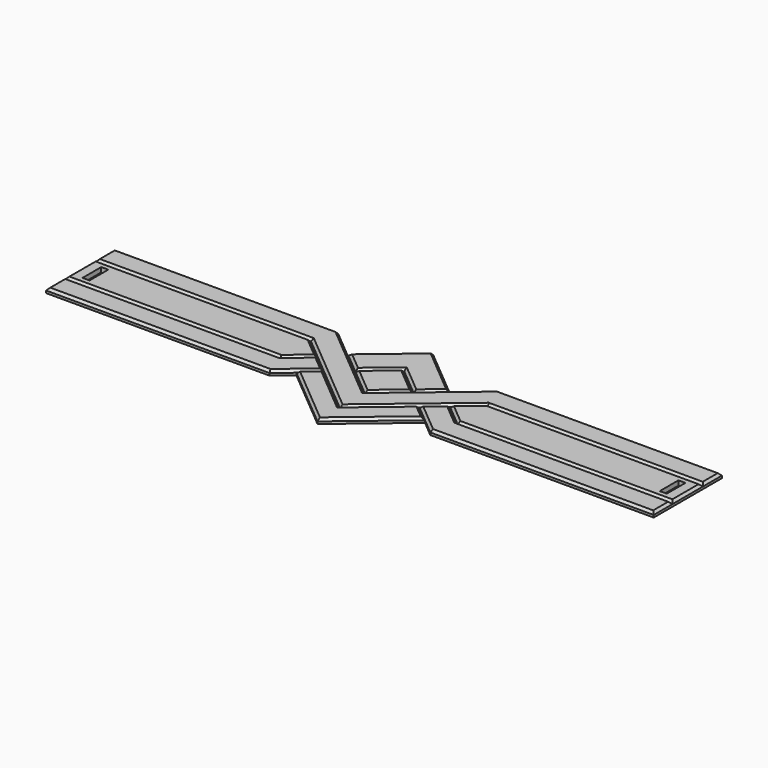
from build123d import *

# Parameters (mm, degrees)
F1_DEPTH  = 2
F3_DEPTH  = 2
F5_DEPTH  = 2
F7_DEPTH  = 2
F9_DEPTH  = 1
F10_SIZE  = 0.99999
F11_W     = 3
F11_H     = 10
F12_DEPTH = 2


# Not quite as in the source:
# - a fillet or chamfer is up to 0.001 mm smaller than in the source, because OpenCascade refuses the exact size


with BuildPart() as f1:
    # F0 (on Top) → F1 (new body)
    with BuildSketch(Plane.XY):
        Polygon((37.9150851114, 8), (28.3810563706, 0), (37.9150851114, -8), (130, -8), (130, 0), (130, 8), align=None)
    extrude(amount=F1_DEPTH)



with BuildPart() as f1b:
    # F0 (on Top) → F1, piece 2 (new body)
    with BuildSketch(Plane.XY):
        Polygon((-37.9150851114, -8), (-28.3810563706, 0), (-37.9150851114, 8), (-130, 8), (-130, 0), (-130, -8), align=None)
    extrude(amount=F1_DEPTH)


with BuildPart() as f3:
    # F2 (on Top) → F3 (new body)
    with BuildSketch(Plane.XY):
        Polygon((-37.8240925528, 8.25), (0, -23.4881821107), (37.8240925528, 8.25), (130, 8.25), (130, 18.25), (34.1843902102, 18.25), (0, -10.4341092174), (-34.1843902102, 18.25), (-130, 18.25), (-130, 8.25), align=None)
    extrude(amount=F3_DEPTH)


with BuildPart() as f5:
    # F4 (on Top) → F5 (new body)
    with BuildSketch(Plane.XY):
        Polygon((12.4810478052, 0.365085215), (21.6735811226, 8.0785365312), (0, 26.2648304575), (-21.6735811226, 8.0785365312), (-12.4810478052, 0.365085215), (0, 10.8379278251), align=None)
    extrude(amount=F5_DEPTH)


with BuildPart() as f5b:
    # F4 (on Top) → F5, piece 2 (new body)
    with BuildSketch(Plane.XY):
        Polygon((37.8240925528, -8.25), (28.1865908923, -0.1631759112), (20.5261464611, -6.591052008), (34.4207396164, -18.25), (130, -18.25), (130, -8.25), align=None)
    extrude(amount=F5_DEPTH)


with BuildPart() as f5c:
    # F4 (on Top) → F5, piece 3 (new body)
    with BuildSketch(Plane.XY):
        Polygon((-130, -18.25), (-34.4207396164, -18.25), (-20.5261464611, -6.591052008), (-28.1865908923, -0.1631759112), (-37.8240925528, -8.25), (-130, -8.25), align=None)
    extrude(amount=F5_DEPTH)


with BuildPart() as f7:
    # F6 (on Top) → F7 (new body)
    with BuildSketch(Plane.XY):
        Polygon((-27.3324382036, -12.6285607212), (0, -35.563199537), (27.3324382036, -12.6285607212), (20.3316809827, -6.7542279192), (0, -23.814533933), (-20.3316809827, -6.7542279192), align=None)
    extrude(amount=F7_DEPTH)


with BuildPart() as f7b:
    # F6 (on Top) → F7, piece 2 (new body)
    with BuildSketch(Plane.XY):
        Polygon((-12.2865823268, 0.2019093038), (0, -10.107757395), (12.2865823268, 0.2019093038), (0, 10.5115760027), align=None)
    extrude(amount=F7_DEPTH)


with BuildPart() as f1_1:
    add(f1.part)

    add(f1b.part)  # F9 merges F1b

    add(f3.part)  # F9 merges F3

    add(f5.part)  # F9 merges F5

    add(f5b.part)  # F9 merges F5b

    add(f5c.part)  # F9 merges F5c

    add(f7.part)  # F9 merges F7

    add(f7b.part)  # F9 merges F7b
    # F8 (on Top) → F9 (join)
    with BuildSketch(Plane.XY):
        Polygon((21.868046601, 7.9153606201), (0, 26.2648304575), (-21.868046601, 7.9153606201), (-34.1843902102, 18.25), (-130, 18.25), (-130, -18.25), (-34.4207396164, -18.25), (-27.526903682, -12.46538481), (0, -35.563199537), (27.526903682, -12.46538481), (34.4207396164, -18.25), (130, -18.25), (130, 18.25), (34.1843902102, 18.25), align=None)
    extrude(amount=F9_DEPTH)

    # F10 (size 1 in the source; OpenCascade refuses exactly that, so slightly less here)
    f10_edges = [f1_1.edges().sort_by_distance(p)[0] for p in [
        (-18.912046, -7.619091, 2),
        (18.912046, -7.619091, 2),
        (83.912046, 8.25, 2),
        (130, 13.25, 2),
        (82.092195, 18.25, 2),
        (17.092195, 3.907945, 2),
        (-17.092195, 3.907945, 2),
        (-82.092195, 18.25, 2),
        (-130, 13.25, 2),
        (-83.912046, 8.25, 2),
        (-33.148071, -4, 2),
        (-33.148071, 4, 2),
        (-83.957543, 8, 2),
        (-130, 0, 2),
        (-83.957543, -8, 2),
        (-83.912046, -8.25, 2),
        (-130, -13.25, 2),
        (-82.21037, -18.25, 2),
        (-27.473443, -12.420526, 2),
        (-24.356369, -3.377114, 2),
        (-33.005342, -4.206588, 2),
        (6.240524, 5.601507, 2),
        (17.077314, 4.221811, 2),
        (10.836791, 17.171683, 2),
        (-10.836791, 17.171683, 2),
        (-17.077314, 4.221811, 2),
        (-6.240524, 5.601507, 2),
        (-6.143291, -4.952924, 2),
        (6.143291, -4.952924, 2),
        (6.143291, 5.356743, 2),
        (-6.143291, 5.356743, 2),
        (-23.83206, -9.691394, 2),
        (-13.666219, -24.09588, 2),
        (13.666219, -24.09588, 2),
        (23.83206, -9.691394, 2),
        (10.16584, -15.284381, 2),
        (-10.16584, -15.284381, 2),
        (33.005342, -4.206588, 2),
        (24.356369, -3.377114, 2),
        (27.473443, -12.420526, 2),
        (82.21037, -18.25, 2),
        (130, -13.25, 2),
        (83.912046, -8.25, 2),
        (33.148071, 4, 2),
        (33.148071, -4, 2),
        (83.957543, -8, 2),
        (130, 0, 2),
        (83.957543, 8, 2),
    ]]
    chamfer(f10_edges, length=F10_SIZE)

    # F11 (on face) → F12 (cut, through all)
    with BuildSketch(Plane.XY.offset(2)):
        with Locations((123.5, 0)):
            Rectangle(F11_W, F11_H)
        with Locations((-123.5, 0)):
            Rectangle(F11_W, F11_H)
    extrude(amount=-F12_DEPTH, mode=Mode.SUBTRACT)


solid = f1_1.part
